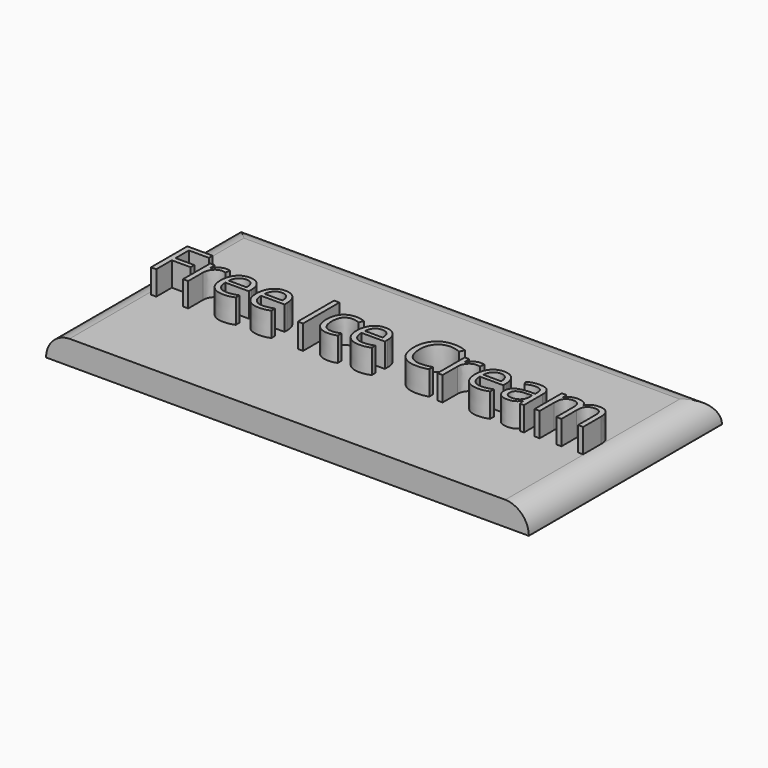
from build123d import *

# Parameters (mm, degrees)
F0_W         = 20
F0_H         = 10
F1_DEPTH     = 1
F2_TEXT_SIZE = 2.6372138463
F3_DEPTH     = 2
F4_T1_DEPTH  = 15.0048288267
F4_T3_DEPTH  = 25.0048288267
F4_T8_DEPTH  = 15.0048288267


# Not quite as in the source:
# - a fillet or chamfer that OpenCascade refuses, or shapes differently, is made with other operations: its cross-section is extruded or revolved along the edge and cut away or added
# - Text() gives the source's letters only with a copy of the font that has no kerning and outlines rounded to 1/6400 em; it was checked with that copy


with BuildPart() as f1:
    # F0 (on Top) → F1 (new body)
    with BuildSketch(Plane.XY):
        Rectangle(F0_W, F0_H)
    extrude(amount=F1_DEPTH)

    # F2 (on Top) → F3 (join)
    with BuildSketch(Plane.XY):
        with Locations((-9.1575463302, -0.9445734322)):
            Text('Free Ice Cream', F2_TEXT_SIZE, font='Open Sans', text_align=(TextAlign.LEFT, TextAlign.BOTTOM))
    extrude(amount=F3_DEPTH)

    # F4: fillet of radius 1 on 3 edges, made by hand

    # F4_s2 → F4_t1 (cut)
    with BuildSketch(Plane.XZ.offset(-7.5024144134)):
        with BuildLine():
            ThreePointArc((-10.0004, -0.0009656854), (-9.7071067812, 0.7071067812), (-8.9990343146, 1.0004))
            Line((-8.9990343146, 1.0004), (-8.9990343146, 1.1005365685))
            ThreePointArc((-8.9990343146, 1.1005365685), (-9.4995171573, 1.1001365685), (-10, 1.1001365685))
            Line((-10, 1.1001365685), (-10.1001365685, 1))
            ThreePointArc((-10.1001365685, 1), (-10.1001365685, 0.4995171573), (-10.1005365685, -0.0009656854))
            Line((-10.1005365685, -0.0009656854), (-10.0004, -0.0009656854))
        make_face()
    extrude(amount=F4_T1_DEPTH, mode=Mode.SUBTRACT)

    # F4_s4 → F4_t3 (cut)
    with BuildSketch(Plane.YZ.offset(-12.5024144134)):
        with BuildLine():
            ThreePointArc((3.9990343146, 1.0004), (4.7071067812, 0.7071067812), (5.0004, -0.0009656854))
            Line((5.0004, -0.0009656854), (5.1005365685, -0.0009656854))
            ThreePointArc((5.1005365685, -0.0009656854), (5.1001365685, 0.4995171573), (5.1001365685, 1))
            Line((5.1001365685, 1), (5, 1.1001365685))
            ThreePointArc((5, 1.1001365685), (4.4995171573, 1.1001365685), (3.9990343146, 1.1005365685))
            Line((3.9990343146, 1.1005365685), (3.9990343146, 1.0004))
        make_face()
    extrude(amount=F4_T3_DEPTH, mode=Mode.SUBTRACT)


with BuildPart() as f4_tool6:
    # F4_s7 → F4_t8 (new body)
    with BuildSketch(Plane.XZ.offset(7.5024144134)):
        with BuildLine():
            ThreePointArc((10.0004, -0.0009656854), (9.7071067812, 0.7071067812), (8.9990343146, 1.0004))
            Line((8.9990343146, 1.0004), (8.9990343146, 1.1005365685))
            ThreePointArc((8.9990343146, 1.1005365685), (9.4995171573, 1.1001365685), (10, 1.1001365685))
            Line((10, 1.1001365685), (10.1001365685, 1))
            ThreePointArc((10.1001365685, 1), (10.1001365685, 0.4995171573), (10.1005365685, -0.0009656854))
            Line((10.1005365685, -0.0009656854), (10.0004, -0.0009656854))
        make_face()
    extrude(amount=-F4_T8_DEPTH)

    split(bisect_by=Plane.YZ.offset(9.0066761005), keep=Keep.TOP)


with BuildPart() as f1_1:
    add(f1.part)

    # F4_t5: cut F4_tool6
    add(f4_tool6.part, mode=Mode.SUBTRACT)


solid = f1_1.part
